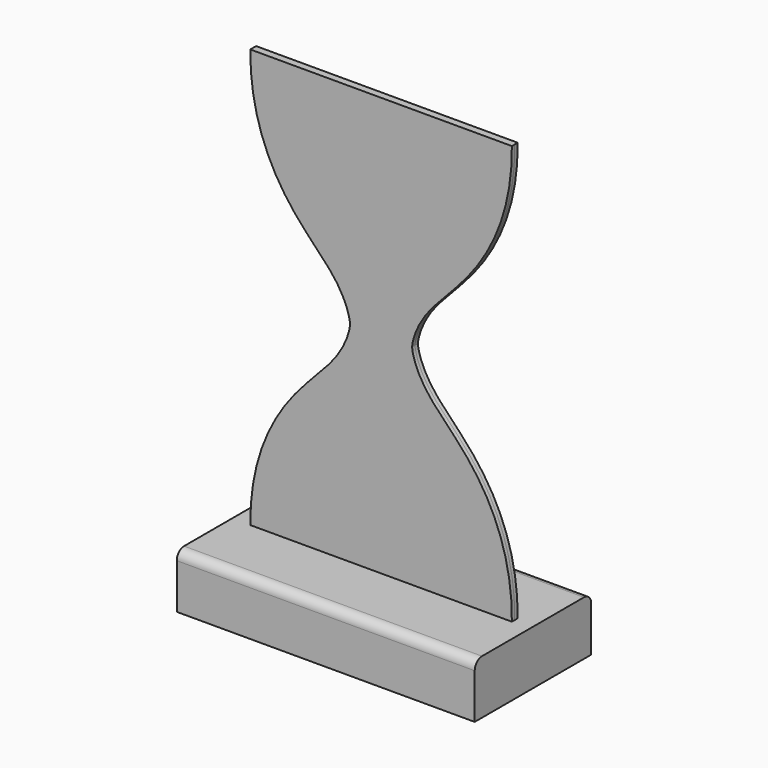
from build123d import *

# Parameters (mm, degrees)
F0_W     = 125.702098012
F0_H     = 18.2329118252
F1_DEPTH = 2
F3_W     = 163.6505723
F3_H     = 29.7609269619
F4_DEPTH = 40
F8_R     = 5


# Not quite as in the source:
# - the program builds the solid bodies; features that only make, move or delete a surface that nothing else refers to are left out


with BuildPart() as f1:
    # F0 (on Front) → F1 (new body, symmetric)
    with BuildSketch(Plane.XZ):
        with BuildLine():
            Line((71.8356221218, 115), (-71.8356221218, 115))
            add(Edge.make_bspline(
                [(-71.8356221218, 115), (-72.1203169337, 82.5445248846), (-52.4850086356, 44.7487745495), (-24.5321077683, 21.5541787538), (-17.5291927784, 5.6703685242), (-17.0137044211, 0)],
                knots=[0, 0, 0, 0, 0.4524273346, 0.7614820627, 1, 1, 1, 1], degree=3))
            add(Edge.make_bspline(
                [(-71.8356221218, -115), (-72.1203169337, -82.5445248846), (-52.4850086356, -44.7487745495), (-24.5321077683, -21.5541787538), (-17.5291927784, -5.6703685242), (-17.0137044211, 0)],
                knots=[0, 0, 0, 0, 0.4524273346, 0.7614820627, 1, 1, 1, 1], degree=3))
            Line((-71.8356221218, -115), (-62.851049006, -115))
            Line((-62.851049006, -115), (62.851049006, -115))
            Line((62.851049006, -115), (71.8356221218, -115))
            add(Edge.make_bspline(
                [(71.8356221218, -115), (72.1203169337, -82.5445248846), (52.4850086356, -44.7487745495), (24.5321077683, -21.5541787538), (17.5291927784, -5.6703685242), (17.0137044211, 0)],
                knots=[0, 0, 0, 0, 0.4524273346, 0.7614820627, 1, 1, 1, 1], degree=3))
            add(Edge.make_bspline(
                [(71.8356221218, 115), (72.1203169337, 82.5445248846), (52.4850086356, 44.7487745495), (24.5321077683, 21.5541787538), (17.5291927784, 5.6703685242), (17.0137044211, 0)],
                knots=[0, 0, 0, 0, 0.4524273346, 0.7614820627, 1, 1, 1, 1], degree=3))
        make_face()
        with Locations((0, -124.1164559126)):
            Rectangle(F0_W, F0_H)
    extrude(amount=F1_DEPTH, both=True)


with BuildPart() as f4:
    # F3 (on Front) → F4 (new body, symmetric)
    with BuildSketch(Plane.XZ):
        with Locations((0, -129.8804634809)):
            Rectangle(F3_W, F3_H)
    extrude(amount=F4_DEPTH, both=True)

    # F5: cut F1
    add(f1.part, mode=Mode.SUBTRACT)

    # F8
    f8_edges = [f4.edges().sort_by_distance(p)[0] for p in [
        (0, -40, -115),
        (0, 40, -115),
    ]]
    fillet(f8_edges, radius=F8_R)


solid = Compound([f1.part, f4.part])
